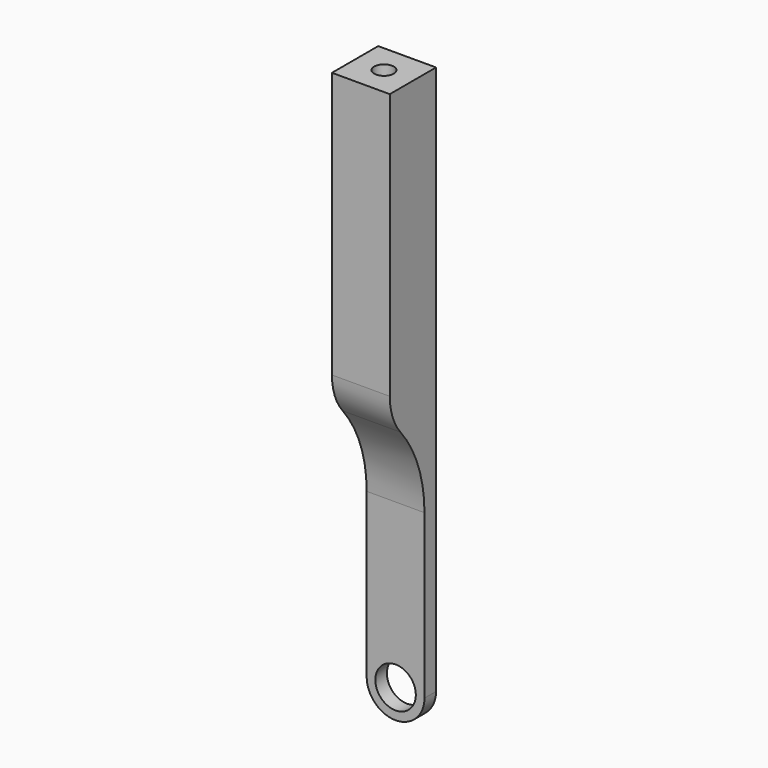
from build123d import *

# Parameters (mm, degrees)
F0_W        = 20
F0_H        = 200
F1_DEPTH    = 20
F2_W        = 15
F2_H        = 100
F3_DEPTH    = 20
F6_R        = 7
F7_DEPTH    = 20.001
F8_T1_DEPTH = 20
F9_R        = 20
F11_D       = 6.7564
F11_DEPTH   = 50
F11_TIP     = 2.0298273432


# Not quite as in the source:
# - a fillet or chamfer that OpenCascade refuses, or shapes differently, is made with other operations: its cross-section is extruded or revolved along the edge and cut away or added


with BuildPart() as f1:
    # F0 (on Front) → F1 (new body)
    with BuildSketch(Plane.XZ):
        with Locations((10, 100)):
            Rectangle(F0_W, F0_H)
    extrude(amount=F1_DEPTH)

    # F2 (on face) → F3 (cut)
    with BuildSketch(Plane.YZ.offset(20)):
        with Locations((-12.5, 50)):
            Rectangle(F2_W, F2_H)
    extrude(amount=-F3_DEPTH, mode=Mode.SUBTRACT)

    # F5: sweep along a path in F5_path
    with BuildLine(Plane(origin=(0, -5, 0), x_dir=(0, -1, 0), z_dir=(0, 0, -1))) as f5_path:
        Line((0, 0), (-5, 0))
    # F4 (on face) → F5 (sweep, cut)
    with BuildSketch(Plane(origin=(0, 0, 0), x_dir=(-1, 0, 0), z_dir=(0, 1, 0))):
        with BuildLine():
            Line((0, 0), (0, 10))
            ThreePointArc((0, 10), (-2.9289321881, 2.9289321881), (-10, 0))
            Line((-10, 0), (0, 0))
        make_face()
        with BuildLine():
            ThreePointArc((-10, 0), (-17.0710678277, 2.9289322039), (-20, 10.0000000447))
            Line((-20, 10.0000000447), (-20, 0))
            Line((-20, 0), (-10, 0))
        make_face()
    sweep(path=f5_path.line, mode=Mode.SUBTRACT)

    # F6 (on face) → F7 (cut, through all)
    with BuildSketch(Plane(origin=(0, 0, 0), x_dir=(-1, 0, 0), z_dir=(0, 1, 0))):
        with Locations((-10, 10)):
            Circle(F6_R)
    extrude(amount=-F7_DEPTH, mode=Mode.SUBTRACT)

    # F8: fillet of radius 45 on 1 edges, made by hand

    # F8_s2 → F8_t1 (join)
    with BuildSketch(Plane.YZ):
        with BuildLine():
            ThreePointArc((-5, 66.4589803375), (-8.9208081871, 84.8301534084), (-20, 100))
            Line((-20, 100), (-5, 100))
            Line((-5, 100), (-5, 66.4589803375))
        make_face()
    extrude(amount=F8_T1_DEPTH)

    # F9
    f9_edges = [f1.edges().sort_by_distance(p)[0] for p in [
        (10, -20, 100),
    ]]
    fillet(f9_edges, radius=F9_R)

    # F11
    with Locations(Plane.XY.offset(200)):
        with Locations((10, -10)):
            Hole(F11_D / 2, depth=F11_DEPTH)
            with Locations((0, 0, -(F11_DEPTH + F11_TIP / 2))):  # 118° drill point
                Cone(0, F11_D / 2, F11_TIP, mode=Mode.SUBTRACT)


solid = f1.part
